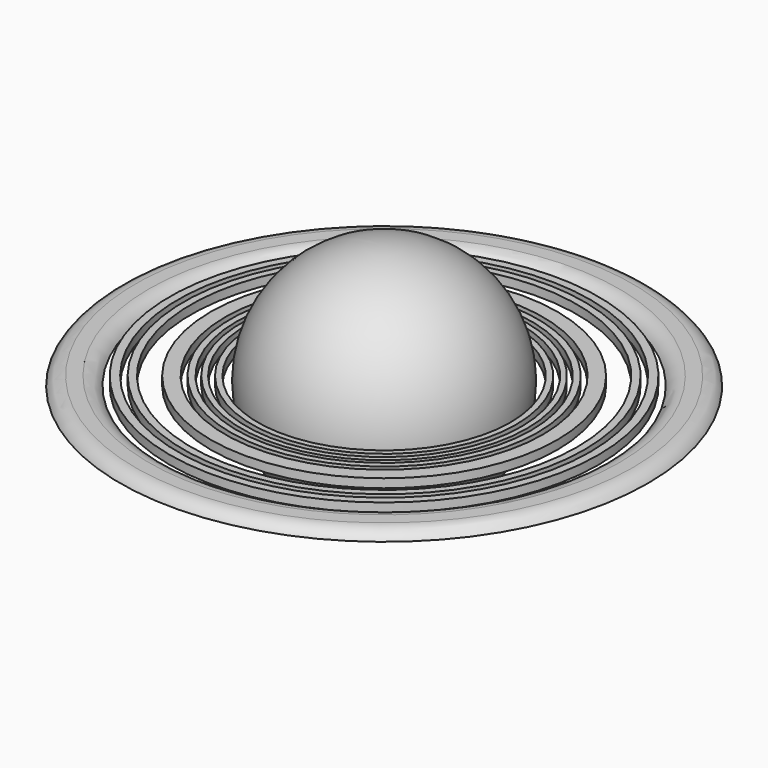
from build123d import *

# Parameters (mm, degrees)
F3_R     = 76.2
F3_R_2   = 63.5
F4_DEPTH = 1.27
F3_R_3   = 61.8612612332
F3_R_4   = 59.512366358
F3_R_5   = 57.8207462115
F3_R_6   = 55.7278531971
F3_R_7   = 50.0426111079
F3_R_8   = 45.8863707971
F3_R_9   = 44.3352929458
F3_R_10  = 42.5414160934
F3_R_11  = 41.2380044226
F3_R_12  = 39.683753914
F3_R_13  = 38.1309941729
F3_R_14  = 36.4646412836


# Not quite as in the source:
# - a fillet or chamfer that OpenCascade refuses, or shapes differently, is made with other operations: its cross-section is extruded or revolved along the edge and cut away or added


with BuildPart() as f2:
    # F0 (on Front) → F2 (revolve)
    with BuildSketch(Plane.XZ):
        with BuildLine():
            Line((0, -34.29), (0, 34.29))
            ThreePointArc((0, 34.29), (-34.29, 0), (0, -34.29))
        make_face()
    revolve(axis=Axis((0, 0, 0), (0, 0, 1)))


with BuildPart() as f4:
    # F3 (on Top) → F4 (new body, symmetric)
    with BuildSketch(Plane.XY):
        Circle(F3_R)
        Circle(F3_R_2, mode=Mode.SUBTRACT)
    extrude(amount=F4_DEPTH, both=True)

    # F5: fillet of radius 5.08 on 2 edges, made by hand

    # F5_s1 → F5_t2 (revolve, cut)
    with BuildSketch(Plane.XZ):
        with BuildLine():
            ThreePointArc((76.2, -1.27), (74.3405909488, 0.5894090512), (71.8005909488, 1.27))
            Line((71.8005909488, 1.27), (76.2, 1.27))
            Line((76.2, 1.27), (76.2, -1.27))
        make_face()
    revolve(axis=Axis((0, 0, 1.27), (0, 0, 1)), mode=Mode.SUBTRACT)

    # F5_s3 → F5_t4 (revolve, cut)
    with BuildSketch(Plane.XZ):
        with BuildLine():
            ThreePointArc((67.8994090512, 1.27), (65.3594090512, 0.5894090512), (63.5, -1.27))
            Line((63.5, -1.27), (63.5, 1.27))
            Line((63.5, 1.27), (67.8994090512, 1.27))
        make_face()
    revolve(axis=Axis((0, 0, 1.27), (0, 0, 1)), mode=Mode.SUBTRACT)


with BuildPart() as f4b:
    # F3 (on Top) → F4, piece 2 (new body, symmetric)
    with BuildSketch(Plane.XY):
        Circle(F3_R_3)
        Circle(F3_R_4, mode=Mode.SUBTRACT)
    extrude(amount=F4_DEPTH, both=True)


with BuildPart() as f4c:
    # F3 (on Top) → F4, piece 3 (new body, symmetric)
    with BuildSketch(Plane.XY):
        Circle(F3_R_5)
        Circle(F3_R_6, mode=Mode.SUBTRACT)
    extrude(amount=F4_DEPTH, both=True)


with BuildPart() as f4d:
    # F3 (on Top) → F4, piece 4 (new body, symmetric)
    with BuildSketch(Plane.XY):
        Circle(F3_R_7)
        Circle(F3_R_8, mode=Mode.SUBTRACT)
    extrude(amount=F4_DEPTH, both=True)


with BuildPart() as f4e:
    # F3 (on Top) → F4, piece 5 (new body, symmetric)
    with BuildSketch(Plane.XY):
        Circle(F3_R_9)
        Circle(F3_R_10, mode=Mode.SUBTRACT)
    extrude(amount=F4_DEPTH, both=True)


with BuildPart() as f4f:
    # F3 (on Top) → F4, piece 6 (new body, symmetric)
    with BuildSketch(Plane.XY):
        Circle(F3_R_11)
        Circle(F3_R_12, mode=Mode.SUBTRACT)
    extrude(amount=F4_DEPTH, both=True)


with BuildPart() as f4g:
    # F3 (on Top) → F4, piece 7 (new body, symmetric)
    with BuildSketch(Plane.XY):
        Circle(F3_R_13)
        Circle(F3_R_14, mode=Mode.SUBTRACT)
    extrude(amount=F4_DEPTH, both=True)


solid = Compound([f2.part, f4.part, f4b.part, f4c.part, f4d.part, f4e.part, f4f.part, f4g.part])
